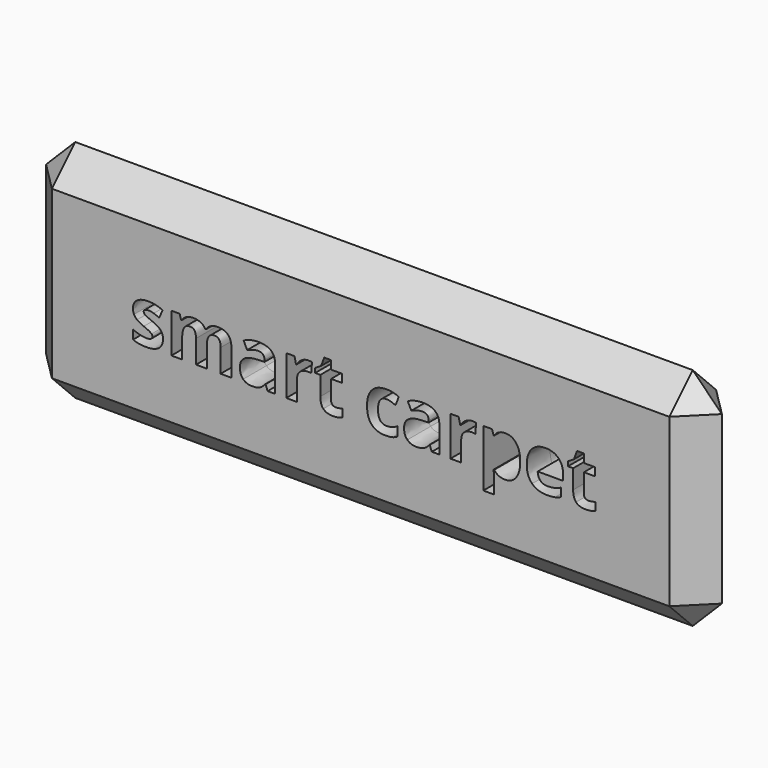
from build123d import *

# Parameters (mm, degrees)
F0_W     = 115.5963391066
F0_H     = 38.5321122594
F1_DEPTH = 5
F2_SIZE  = 4.99999


# Not quite as in the source:
# - a fillet or chamfer is up to 0.001 mm smaller than in the source, because OpenCascade refuses the exact size


with BuildPart() as f1:
    # F0 (on Front) → F1 (new body, symmetric)
    with BuildSketch(Plane.XZ):
        with Locations((0, 2.1674314048)):
            Rectangle(F0_W, F0_H)
        with BuildLine():
            add(Edge.make_bspline(
                [(-33.978614819, 0.8299154837), (-33.8024505908, 0.4669397388), (-33.8024505908, -0.0344507568)],
                knots=[0, 0, 0, 1, 1, 1], degree=2))
            add(Edge.make_bspline(
                [(-33.8024505908, -0.0344507568), (-33.8024505908, -1.0759491607), (-34.5254982746, -1.6208967457)],
                knots=[0, 0, 0, 1, 1, 1], degree=2))
            add(Edge.make_bspline(
                [(-34.5254982746, -1.6208967457), (-35.2485459583, -2.1658443306), (-36.688833714, -2.1658443306)],
                knots=[0, 0, 0, 1, 1, 1], degree=2))
            add(Edge.make_bspline(
                [(-36.688833714, -2.1658443306), (-37.4264004275, -2.1658443306), (-37.9471496295, -2.0651790574)],
                knots=[0, 0, 0, 1, 1, 1], degree=2))
            add(Edge.make_bspline(
                [(-37.9471496295, -2.0651790574), (-38.4678988315, -1.9645137842), (-38.9208925611, -1.7709267202)],
                knots=[0, 0, 0, 1, 1, 1], degree=2))
            Line((-38.9208925611, -1.7709267202), (-38.9208925611, -0.2473965271))
            add(Edge.make_bspline(
                [(-38.9208925611, -0.2473965271), (-38.4078868417, -0.489380357), (-37.7632419188, -0.652961426)],
                knots=[0, 0, 0, 1, 1, 1], degree=2))
            add(Edge.make_bspline(
                [(-37.7632419188, -0.652961426), (-37.1185969959, -0.8165424951), (-36.6288217242, -0.8165424951)],
                knots=[0, 0, 0, 1, 1, 1], degree=2))
            add(Edge.make_bspline(
                [(-36.6288217242, -0.8165424951), (-35.6241048624, -0.8165424951), (-35.6241048624, -0.2357813033)],
                knots=[0, 0, 0, 1, 1, 1], degree=2))
            add(Edge.make_bspline(
                [(-35.6241048624, -0.2357813033), (-35.6241048624, -0.017027921), (-35.7576799365, 0.119450959)],
                knots=[0, 0, 0, 1, 1, 1], degree=2))
            add(Edge.make_bspline(
                [(-35.7576799365, 0.119450959), (-35.8912550106, 0.2559298391), (-36.2174492133, 0.428222326)],
                knots=[0, 0, 0, 1, 1, 1], degree=2))
            add(Edge.make_bspline(
                [(-36.2174492133, 0.428222326), (-36.543643416, 0.6005148129), (-37.0876230657, 0.8289475483)],
                knots=[0, 0, 0, 1, 1, 1], degree=2))
            add(Edge.make_bspline(
                [(-37.0876230657, 0.8289475483), (-37.8677789333, 1.1561096864), (-38.2346264195, 1.4348750584)],
                knots=[0, 0, 0, 1, 1, 1], degree=2))
            add(Edge.make_bspline(
                [(-38.2346264195, 1.4348750584), (-38.6014739056, 1.7136404305), (-38.7669908453, 2.0737123694)],
                knots=[0, 0, 0, 1, 1, 1], degree=2))
            add(Edge.make_bspline(
                [(-38.7669908453, 2.0737123694), (-38.9325077849, 2.4337843083), (-38.9325077849, 2.9584052516)],
                knots=[0, 0, 0, 1, 1, 1], degree=2))
            add(Edge.make_bspline(
                [(-38.9325077849, 2.9584052516), (-38.9325077849, 3.8605209695), (-38.2346264195, 4.3532000472)],
                knots=[0, 0, 0, 1, 1, 1], degree=2))
            add(Edge.make_bspline(
                [(-38.2346264195, 4.3532000472), (-37.536745054, 4.8458791249), (-36.2532628201, 4.8458791249)],
                knots=[0, 0, 0, 1, 1, 1], degree=2))
            add(Edge.make_bspline(
                [(-36.2532628201, 4.8458791249), (-35.0317284467, 4.8458791249), (-33.8760136751, 4.3135146991)],
                knots=[0, 0, 0, 1, 1, 1], degree=2))
            Line((-33.8760136751, 4.3135146991), (-34.4316085486, 2.9835715699))
            add(Edge.make_bspline(
                [(-34.4316085486, 2.9835715699), (-34.9407425267, 3.2003890815), (-35.3821210324, 3.3397717675)],
                knots=[0, 0, 0, 1, 1, 1], degree=2))
            add(Edge.make_bspline(
                [(-35.3821210324, 3.3397717675), (-35.8234995382, 3.4791544535), (-36.2842367504, 3.4791544535)],
                knots=[0, 0, 0, 1, 1, 1], degree=2))
            add(Edge.make_bspline(
                [(-36.2842367504, 3.4791544535), (-37.1011741601, 3.4791544535), (-37.1011741601, 3.0377759478)],
                knots=[0, 0, 0, 1, 1, 1], degree=2))
            add(Edge.make_bspline(
                [(-37.1011741601, 3.0377759478), (-37.1011741601, 2.789984506), (-36.8378957532, 2.6080126659)],
                knots=[0, 0, 0, 1, 1, 1], degree=2))
            add(Edge.make_bspline(
                [(-36.8378957532, 2.6080126659), (-36.5746173463, 2.4260408258), (-35.6841168522, 2.0698406281)],
                knots=[0, 0, 0, 1, 1, 1], degree=2))
            add(Edge.make_bspline(
                [(-35.6841168522, 2.0698406281), (-34.8923457607, 1.748486102), (-34.5235624039, 1.4706886653)],
                knots=[0, 0, 0, 1, 1, 1], degree=2))
            add(Edge.make_bspline(
                [(-34.5235624039, 1.4706886653), (-34.1547790471, 1.1928912285), (-33.978614819, 0.8299154837)],
                knots=[0, 0, 0, 1, 1, 1], degree=2))
        make_face(mode=Mode.SUBTRACT)
        with BuildLine():
            Line((-26.3086953461, 1.3496967503), (-26.3086953461, -2.0438844804))
            Line((-26.3086953461, -2.0438844804), (-28.1535800653, -2.0438844804))
            Line((-28.1535800653, -2.0438844804), (-28.1535800653, 1.9072274944))
            add(Edge.make_bspline(
                [(-28.1535800653, 1.9072274944), (-28.1535800653, 2.6389865961), (-28.3984677012, 3.0048661469)],
                knots=[0, 0, 0, 1, 1, 1], degree=2))
            add(Edge.make_bspline(
                [(-28.3984677012, 3.0048661469), (-28.6433553371, 3.3707456977), (-29.1699121509, 3.3707456977)],
                knots=[0, 0, 0, 1, 1, 1], degree=2))
            add(Edge.make_bspline(
                [(-29.1699121509, 3.3707456977), (-29.8784408049, 3.3707456977), (-30.1988273957, 2.8499964958)],
                knots=[0, 0, 0, 1, 1, 1], degree=2))
            add(Edge.make_bspline(
                [(-30.1988273957, 2.8499964958), (-30.5192139865, 2.3292472938), (-30.5192139865, 1.1386868506)],
                knots=[0, 0, 0, 1, 1, 1], degree=2))
            Line((-30.5192139865, 1.1386868506), (-30.5192139865, -2.0438844804))
            Line((-30.5192139865, -2.0438844804), (-32.3640987058, -2.0438844804))
            Line((-32.3640987058, -2.0438844804), (-32.3640987058, 4.7200475333))
            Line((-32.3640987058, 4.7200475333), (-30.9547848804, 4.7200475333))
            Line((-30.9547848804, 4.7200475333), (-30.7069934385, 3.8547133576))
            Line((-30.7069934385, 3.8547133576), (-30.6043922947, 3.8547133576))
            add(Edge.make_bspline(
                [(-30.6043922947, 3.8547133576), (-30.3314345345, 4.3212581816), (-29.8174608798, 4.5835686533)],
                knots=[0, 0, 0, 1, 1, 1], degree=2))
            add(Edge.make_bspline(
                [(-29.8174608798, 4.5835686533), (-29.3034872251, 4.8458791249), (-28.6375477251, 4.8458791249)],
                knots=[0, 0, 0, 1, 1, 1], degree=2))
            add(Edge.make_bspline(
                [(-28.6375477251, 4.8458791249), (-27.1198251439, 4.8458791249), (-26.5797172356, 3.8547133576)],
                knots=[0, 0, 0, 1, 1, 1], degree=2))
            Line((-26.5797172356, 3.8547133576), (-26.4171041019, 3.8547133576))
            add(Edge.make_bspline(
                [(-26.4171041019, 3.8547133576), (-26.1441463417, 4.3270657936), (-25.6156536572, 4.5864724592)],
                knots=[0, 0, 0, 1, 1, 1], degree=2))
            add(Edge.make_bspline(
                [(-25.6156536572, 4.5864724592), (-25.0871609727, 4.8458791249), (-24.4212214727, 4.8458791249)],
                knots=[0, 0, 0, 1, 1, 1], degree=2))
            add(Edge.make_bspline(
                [(-24.4212214727, 4.8458791249), (-23.271314313, 4.8458791249), (-22.6818417033, 4.2564065152)],
                knots=[0, 0, 0, 1, 1, 1], degree=2))
            add(Edge.make_bspline(
                [(-22.6818417033, 4.2564065152), (-22.0923690937, 3.6669339056), (-22.0923690937, 2.3660288359)],
                knots=[0, 0, 0, 1, 1, 1], degree=2))
            Line((-22.0923690937, 2.3660288359), (-22.0923690937, -2.0438844804))
            Line((-22.0923690937, -2.0438844804), (-23.9430614248, -2.0438844804))
            Line((-23.9430614248, -2.0438844804), (-23.9430614248, 1.9072274944))
            add(Edge.make_bspline(
                [(-23.9430614248, 1.9072274944), (-23.9430614248, 2.6389865961), (-24.1879490607, 3.0048661469)],
                knots=[0, 0, 0, 1, 1, 1], degree=2))
            add(Edge.make_bspline(
                [(-24.1879490607, 3.0048661469), (-24.4328366966, 3.3707456977), (-24.9593935105, 3.3707456977)],
                knots=[0, 0, 0, 1, 1, 1], degree=2))
            add(Edge.make_bspline(
                [(-24.9593935105, 3.3707456977), (-25.6369482342, 3.3707456977), (-25.9728217901, 2.8867780379)],
                knots=[0, 0, 0, 1, 1, 1], degree=2))
            add(Edge.make_bspline(
                [(-25.9728217901, 2.8867780379), (-26.3086953461, 2.4028103781), (-26.3086953461, 1.3496967503)],
                knots=[0, 0, 0, 1, 1, 1], degree=2))
        make_face(mode=Mode.SUBTRACT)
        with BuildLine():
            Line((-14.6160366847, -2.0438844804), (-15.9033906598, -2.0438844804))
            Line((-15.9033906598, -2.0438844804), (-16.2615267281, -1.1243459267))
            Line((-16.2615267281, -1.1243459267), (-16.3099234941, -1.1243459267))
            add(Edge.make_bspline(
                [(-16.3099234941, -1.1243459267), (-16.7745324475, -1.7109147304), (-17.2681794605, -1.9383795305)],
                knots=[0, 0, 0, 1, 1, 1], degree=2))
            add(Edge.make_bspline(
                [(-17.2681794605, -1.9383795305), (-17.7618264736, -2.1658443306), (-18.553597565, -2.1658443306)],
                knots=[0, 0, 0, 1, 1, 1], degree=2))
            add(Edge.make_bspline(
                [(-18.553597565, -2.1658443306), (-19.5273404966, -2.1658443306), (-20.0868071114, -1.6083135865)],
                knots=[0, 0, 0, 1, 1, 1], degree=2))
            add(Edge.make_bspline(
                [(-20.0868071114, -1.6083135865), (-20.6462737261, -1.0507828424), (-20.6462737261, -0.0228355329)],
                knots=[0, 0, 0, 1, 1, 1], degree=2))
            add(Edge.make_bspline(
                [(-20.6462737261, -0.0228355329), (-20.6462737261, 1.0535085425), (-19.8932200474, 1.5645783913)],
                knots=[0, 0, 0, 1, 1, 1], degree=2))
            add(Edge.make_bspline(
                [(-19.8932200474, 1.5645783913), (-19.1401663687, 2.0756482401), (-17.6224437875, 2.129852618)],
                knots=[0, 0, 0, 1, 1, 1], degree=2))
            Line((-17.6224437875, 2.129852618), (-16.4473703095, 2.1666341601))
            Line((-16.4473703095, 2.1666341601), (-16.4473703095, 2.4628223679))
            add(Edge.make_bspline(
                [(-16.4473703095, 2.4628223679), (-16.4473703095, 3.4907696774), (-17.5004839373, 3.4907696774)],
                knots=[0, 0, 0, 1, 1, 1], degree=2))
            add(Edge.make_bspline(
                [(-17.5004839373, 3.4907696774), (-18.3116137351, 3.4907696774), (-19.407316517, 3.0009944056)],
                knots=[0, 0, 0, 1, 1, 1], degree=2))
            Line((-19.407316517, 3.0009944056), (-20.0171157683, 4.2476950973))
            add(Edge.make_bspline(
                [(-20.0171157683, 4.2476950973), (-18.8497857728, 4.8594302194), (-17.4288567236, 4.8594302194)],
                knots=[0, 0, 0, 1, 1, 1], degree=2))
            add(Edge.make_bspline(
                [(-17.4288567236, 4.8594302194), (-16.0679396642, 4.8594302194), (-15.3419881744, 4.2660858684)],
                knots=[0, 0, 0, 1, 1, 1], degree=2))
            add(Edge.make_bspline(
                [(-15.3419881744, 4.2660858684), (-14.6160366847, 3.6727415175), (-14.6160366847, 2.4628223679)],
                knots=[0, 0, 0, 1, 1, 1], degree=2))
            Line((-14.6160366847, 2.4628223679), (-14.6160366847, -2.0438844804))
        make_face(mode=Mode.SUBTRACT)
        with BuildLine():
            add(Edge.make_bspline(
                [(-10.1044901598, 4.4983903451), (-9.5692219281, 4.8458791249), (-8.9400639703, 4.8458791249)],
                knots=[0, 0, 0, 1, 1, 1], degree=2))
            add(Edge.make_bspline(
                [(-8.9400639703, 4.8458791249), (-8.5645050663, 4.8458791249), (-8.3167136244, 4.791674747)],
                knots=[0, 0, 0, 1, 1, 1], degree=2))
            Line((-8.3167136244, 4.791674747), (-8.4560963105, 3.0629422661))
            add(Edge.make_bspline(
                [(-8.4560963105, 3.0629422661), (-8.6806573046, 3.1229542559), (-9.0000759601, 3.1229542559)],
                knots=[0, 0, 0, 1, 1, 1], degree=2))
            add(Edge.make_bspline(
                [(-9.0000759601, 3.1229542559), (-9.8828329716, 3.1229542559), (-10.3764799846, 2.668992591)],
                knots=[0, 0, 0, 1, 1, 1], degree=2))
            add(Edge.make_bspline(
                [(-10.3764799846, 2.668992591), (-10.8701269977, 2.2150309261), (-10.8701269977, 1.3980935163)],
                knots=[0, 0, 0, 1, 1, 1], degree=2))
            Line((-10.8701269977, 1.3980935163), (-10.8701269977, -2.0438844804))
            Line((-10.8701269977, -2.0438844804), (-12.7150117169, -2.0438844804))
            Line((-12.7150117169, -2.0438844804), (-12.7150117169, 4.7200475333))
            Line((-12.7150117169, 4.7200475333), (-11.3173131153, 4.7200475333))
            Line((-11.3173131153, 4.7200475333), (-11.0443553552, 3.5817555974))
            Line((-11.0443553552, 3.5817555974), (-10.9553053058, 3.5817555974))
            add(Edge.make_bspline(
                [(-10.9553053058, 3.5817555974), (-10.6397583916, 4.1509015654), (-10.1044901598, 4.4983903451)],
                knots=[0, 0, 0, 1, 1, 1], degree=2))
        make_face(mode=Mode.SUBTRACT)
        with BuildLine():
            add(Edge.make_bspline(
                [(-4.8244029911, -0.5068031928), (-4.6037137383, -0.6945826448), (-4.2397700581, -0.6945826448)],
                knots=[0, 0, 0, 1, 1, 1], degree=2))
            add(Edge.make_bspline(
                [(-4.2397700581, -0.6945826448), (-3.7558023982, -0.6945826448), (-3.0782476745, -0.4835727451)],
                knots=[0, 0, 0, 1, 1, 1], degree=2))
            Line((-3.0782476745, -0.4835727451), (-3.0782476745, -1.8561050284))
            add(Edge.make_bspline(
                [(-3.0782476745, -1.8561050284), (-3.7674176221, -2.1658443306), (-4.7721344839, -2.1658443306)],
                knots=[0, 0, 0, 1, 1, 1], degree=2))
            add(Edge.make_bspline(
                [(-4.7721344839, -2.1658443306), (-5.8794524896, -2.1658443306), (-6.3847147264, -1.6054097806)],
                knots=[0, 0, 0, 1, 1, 1], degree=2))
            add(Edge.make_bspline(
                [(-6.3847147264, -1.6054097806), (-6.8899769633, -1.0449752305), (-6.8899769633, 0.073957999)],
                knots=[0, 0, 0, 1, 1, 1], degree=2))
            Line((-6.8899769633, 0.073957999), (-6.8899769633, 3.3339641556))
            Line((-6.8899769633, 3.3339641556), (-7.7727339748, 3.3339641556))
            Line((-7.7727339748, 3.3339641556), (-7.7727339748, 4.1141200232))
            Line((-7.7727339748, 4.1141200232), (-6.7564018892, 4.7316627572))
            Line((-6.7564018892, 4.7316627572), (-6.2240374633, 6.160335289))
            Line((-6.2240374633, 6.160335289), (-5.045092244, 6.160335289))
            Line((-5.045092244, 6.160335289), (-5.045092244, 4.7200475333))
            Line((-5.045092244, 4.7200475333), (-3.1518107588, 4.7200475333))
            Line((-3.1518107588, 4.7200475333), (-3.1518107588, 3.3339641556))
            Line((-3.1518107588, 3.3339641556), (-5.045092244, 3.3339641556))
            Line((-5.045092244, 3.3339641556), (-5.045092244, 0.073957999))
            add(Edge.make_bspline(
                [(-5.045092244, 0.073957999), (-5.045092244, -0.3190237408), (-4.8244029911, -0.5068031928)],
                knots=[0, 0, 0, 1, 1, 1], degree=2))
        make_face(mode=Mode.SUBTRACT)
        with BuildLine():
            add(Edge.make_bspline(
                [(5.4066733375, -2.0564676395), (4.9498078667, -2.1658443306), (4.2548303072, -2.1658443306)],
                knots=[0, 0, 0, 1, 1, 1], degree=2))
            add(Edge.make_bspline(
                [(4.2548303072, -2.1658443306), (1.0974252945, -2.1658443306), (1.0974252945, 1.3012999843)],
                knots=[0, 0, 0, 1, 1, 1], degree=2))
            add(Edge.make_bspline(
                [(1.0974252945, 1.3012999843), (1.0974252945, 3.0261607239), (1.955983923, 3.9360199244)],
                knots=[0, 0, 0, 1, 1, 1], degree=2))
            add(Edge.make_bspline(
                [(1.955983923, 3.9360199244), (2.8145425515, 4.8458791249), (4.4174434409, 4.8458791249)],
                knots=[0, 0, 0, 1, 1, 1], degree=2))
            add(Edge.make_bspline(
                [(4.4174434409, 4.8458791249), (5.5905810483, 4.8458791249), (6.5236706964, 4.3870777834)],
                knots=[0, 0, 0, 1, 1, 1], degree=2))
            Line((6.5236706964, 4.3870777834), (5.9777551761, 2.9584052516))
            add(Edge.make_bspline(
                [(5.9777551761, 2.9584052516), (5.5421842823, 3.1345694797), (5.1675933136, 3.2468499768)],
                knots=[0, 0, 0, 1, 1, 1], degree=2))
            add(Edge.make_bspline(
                [(5.1675933136, 3.2468499768), (4.7930023449, 3.3591304739), (4.4174434409, 3.3591304739)],
                knots=[0, 0, 0, 1, 1, 1], degree=2))
            add(Edge.make_bspline(
                [(4.4174434409, 3.3591304739), (2.9771556852, 3.3591304739), (2.9771556852, 1.3129152082)],
                knots=[0, 0, 0, 1, 1, 1], degree=2))
            add(Edge.make_bspline(
                [(2.9771556852, 1.3129152082), (2.9771556852, -0.6713521971), (4.4174434409, -0.6713521971)],
                knots=[0, 0, 0, 1, 1, 1], degree=2))
            add(Edge.make_bspline(
                [(4.4174434409, -0.6713521971), (4.9498078667, -0.6713521971), (5.4037695316, -0.5290657051)],
                knots=[0, 0, 0, 1, 1, 1], degree=2))
            add(Edge.make_bspline(
                [(5.4037695316, -0.5290657051), (5.8577311965, -0.3867792131), (6.3107249261, -0.0828475228)],
                knots=[0, 0, 0, 1, 1, 1], degree=2))
            Line((6.3107249261, -0.0828475228), (6.3107249261, -1.6625179644))
            add(Edge.make_bspline(
                [(6.3107249261, -1.6625179644), (5.8635388084, -1.9470909484), (5.4066733375, -2.0564676395)],
                knots=[0, 0, 0, 1, 1, 1], degree=2))
        make_face(mode=Mode.SUBTRACT)
        with BuildLine():
            Line((13.4618310677, -2.0438844804), (12.1744770925, -2.0438844804))
            Line((12.1744770925, -2.0438844804), (11.8163410243, -1.1243459267))
            Line((11.8163410243, -1.1243459267), (11.7679442583, -1.1243459267))
            add(Edge.make_bspline(
                [(11.7679442583, -1.1243459267), (11.3033353048, -1.7109147304), (10.8096882918, -1.9383795305)],
                knots=[0, 0, 0, 1, 1, 1], degree=2))
            add(Edge.make_bspline(
                [(10.8096882918, -1.9383795305), (10.3160412788, -2.1658443306), (9.5242701873, -2.1658443306)],
                knots=[0, 0, 0, 1, 1, 1], degree=2))
            add(Edge.make_bspline(
                [(9.5242701873, -2.1658443306), (8.5505272558, -2.1658443306), (7.991060641, -1.6083135865)],
                knots=[0, 0, 0, 1, 1, 1], degree=2))
            add(Edge.make_bspline(
                [(7.991060641, -1.6083135865), (7.4315940263, -1.0507828424), (7.4315940263, -0.0228355329)],
                knots=[0, 0, 0, 1, 1, 1], degree=2))
            add(Edge.make_bspline(
                [(7.4315940263, -0.0228355329), (7.4315940263, 1.0535085425), (8.1846477049, 1.5645783913)],
                knots=[0, 0, 0, 1, 1, 1], degree=2))
            add(Edge.make_bspline(
                [(8.1846477049, 1.5645783913), (8.9377013836, 2.0756482401), (10.4554239648, 2.129852618)],
                knots=[0, 0, 0, 1, 1, 1], degree=2))
            Line((10.4554239648, 2.129852618), (11.6304974429, 2.1666341601))
            Line((11.6304974429, 2.1666341601), (11.6304974429, 2.4628223679))
            add(Edge.make_bspline(
                [(11.6304974429, 2.4628223679), (11.6304974429, 3.4907696774), (10.5773838151, 3.4907696774)],
                knots=[0, 0, 0, 1, 1, 1], degree=2))
            add(Edge.make_bspline(
                [(10.5773838151, 3.4907696774), (9.7662540172, 3.4907696774), (8.6705512354, 3.0009944056)],
                knots=[0, 0, 0, 1, 1, 1], degree=2))
            Line((8.6705512354, 3.0009944056), (8.060751984, 4.2476950973))
            add(Edge.make_bspline(
                [(8.060751984, 4.2476950973), (9.2280819795, 4.8594302194), (10.6490110288, 4.8594302194)],
                knots=[0, 0, 0, 1, 1, 1], degree=2))
            add(Edge.make_bspline(
                [(10.6490110288, 4.8594302194), (12.0099280882, 4.8594302194), (12.7358795779, 4.2660858684)],
                knots=[0, 0, 0, 1, 1, 1], degree=2))
            add(Edge.make_bspline(
                [(12.7358795779, 4.2660858684), (13.4618310677, 3.6727415175), (13.4618310677, 2.4628223679)],
                knots=[0, 0, 0, 1, 1, 1], degree=2))
            Line((13.4618310677, 2.4628223679), (13.4618310677, -2.0438844804))
        make_face(mode=Mode.SUBTRACT)
        with BuildLine():
            add(Edge.make_bspline(
                [(17.9733775925, 4.4983903451), (18.5086458243, 4.8458791249), (19.1378037821, 4.8458791249)],
                knots=[0, 0, 0, 1, 1, 1], degree=2))
            add(Edge.make_bspline(
                [(19.1378037821, 4.8458791249), (19.5133626861, 4.8458791249), (19.7611541279, 4.791674747)],
                knots=[0, 0, 0, 1, 1, 1], degree=2))
            Line((19.7611541279, 4.791674747), (19.6217714419, 3.0629422661))
            add(Edge.make_bspline(
                [(19.6217714419, 3.0629422661), (19.3972104478, 3.1229542559), (19.0777917923, 3.1229542559)],
                knots=[0, 0, 0, 1, 1, 1], degree=2))
            add(Edge.make_bspline(
                [(19.0777917923, 3.1229542559), (18.1950347807, 3.1229542559), (17.7013877677, 2.668992591)],
                knots=[0, 0, 0, 1, 1, 1], degree=2))
            add(Edge.make_bspline(
                [(17.7013877677, 2.668992591), (17.2077407547, 2.2150309261), (17.2077407547, 1.3980935163)],
                knots=[0, 0, 0, 1, 1, 1], degree=2))
            Line((17.2077407547, 1.3980935163), (17.2077407547, -2.0438844804))
            Line((17.2077407547, -2.0438844804), (15.3628560355, -2.0438844804))
            Line((15.3628560355, -2.0438844804), (15.3628560355, 4.7200475333))
            Line((15.3628560355, 4.7200475333), (16.760554637, 4.7200475333))
            Line((16.760554637, 4.7200475333), (17.0335123972, 3.5817555974))
            Line((17.0335123972, 3.5817555974), (17.1225624466, 3.5817555974))
            add(Edge.make_bspline(
                [(17.1225624466, 3.5817555974), (17.4381093608, 4.1509015654), (17.9733775925, 4.4983903451)],
                knots=[0, 0, 0, 1, 1, 1], degree=2))
        make_face(mode=Mode.SUBTRACT)
        with BuildLine():
            add(Edge.make_bspline(
                [(26.0817717652, -1.7476962726), (25.4952029615, -2.1658443306), (24.7034318701, -2.1658443306)],
                knots=[0, 0, 0, 1, 1, 1], degree=2))
            add(Edge.make_bspline(
                [(24.7034318701, -2.1658443306), (23.5109355563, -2.1658443306), (22.8333808325, -1.3005101549)],
                knots=[0, 0, 0, 1, 1, 1], degree=2))
            Line((22.8333808325, -1.3005101549), (22.7365873005, -1.3005101549))
            add(Edge.make_bspline(
                [(22.7365873005, -1.3005101549), (22.8333808325, -2.1464856243), (22.8333808325, -2.2800606984)],
                knots=[0, 0, 0, 1, 1, 1], degree=2))
            Line((22.8333808325, -2.2800606984), (22.8333808325, -5.0212535236))
            Line((22.8333808325, -5.0212535236), (20.9884961133, -5.0212535236))
            Line((20.9884961133, -5.0212535236), (20.9884961133, 4.7200475333))
            Line((20.9884961133, 4.7200475333), (22.4887958587, 4.7200475333))
            Line((22.4887958587, 4.7200475333), (22.7482025244, 3.8430981337))
            Line((22.7482025244, 3.8430981337), (22.8333808325, 3.8430981337))
            add(Edge.make_bspline(
                [(22.8333808325, 3.8430981337), (23.4818974967, 4.8458791249), (24.751828636, 4.8458791249)],
                knots=[0, 0, 0, 1, 1, 1], degree=2))
            add(Edge.make_bspline(
                [(24.751828636, 4.8458791249), (25.9501325618, 4.8458791249), (26.6276872855, 3.9205329593)],
                knots=[0, 0, 0, 1, 1, 1], degree=2))
            add(Edge.make_bspline(
                [(26.6276872855, 3.9205329593), (27.3052420093, 2.9951867937), (27.3052420093, 1.3496967503)],
                knots=[0, 0, 0, 1, 1, 1], degree=2))
            add(Edge.make_bspline(
                [(27.3052420093, 1.3496967503), (27.3052420093, 0.2675450629), (26.9867912891, -0.5310015758)],
                knots=[0, 0, 0, 1, 1, 1], degree=2))
            add(Edge.make_bspline(
                [(26.9867912891, -0.5310015758), (26.668340569, -1.3295482145), (26.0817717652, -1.7476962726)],
                knots=[0, 0, 0, 1, 1, 1], degree=2))
        make_face(mode=Mode.SUBTRACT)
        with BuildLine():
            add(Edge.make_bspline(
                [(33.2328779068, -2.0477562217), (32.6830906453, -2.1658443306), (31.8893836831, -2.1658443306)],
                knots=[0, 0, 0, 1, 1, 1], degree=2))
            add(Edge.make_bspline(
                [(31.8893836831, -2.1658443306), (30.2574447342, -2.1658443306), (29.3379061805, -1.2637286127)],
                knots=[0, 0, 0, 1, 1, 1], degree=2))
            add(Edge.make_bspline(
                [(29.3379061805, -1.2637286127), (28.4183676269, -0.3616128948), (28.4183676269, 1.2896847605)],
                knots=[0, 0, 0, 1, 1, 1], degree=2))
            add(Edge.make_bspline(
                [(28.4183676269, 1.2896847605), (28.4183676269, 2.9893791818), (29.2682148375, 3.9176291533)],
                knots=[0, 0, 0, 1, 1, 1], degree=2))
            add(Edge.make_bspline(
                [(29.2682148375, 3.9176291533), (30.1180620482, 4.8458791249), (31.6183617936, 4.8458791249)],
                knots=[0, 0, 0, 1, 1, 1], degree=2))
            add(Edge.make_bspline(
                [(31.6183617936, 4.8458791249), (33.0509060667, 4.8458791249), (33.8494527054, 4.0299096504)],
                knots=[0, 0, 0, 1, 1, 1], degree=2))
            add(Edge.make_bspline(
                [(33.8494527054, 4.0299096504), (34.6479993441, 3.213940176), (34.6479993441, 1.7736524203)],
                knots=[0, 0, 0, 1, 1, 1], degree=2))
            Line((34.6479993441, 1.7736524203), (34.6479993441, 0.8773443143))
            Line((34.6479993441, 0.8773443143), (30.2864827938, 0.8773443143))
            add(Edge.make_bspline(
                [(30.2864827938, 0.8773443143), (30.317456724, 0.0913808348), (30.7530276179, -0.349997671)],
                knots=[0, 0, 0, 1, 1, 1], degree=2))
            add(Edge.make_bspline(
                [(30.7530276179, -0.349997671), (31.1885985117, -0.7913761767), (31.9745619913, -0.7913761767)],
                knots=[0, 0, 0, 1, 1, 1], degree=2))
            add(Edge.make_bspline(
                [(31.9745619913, -0.7913761767), (32.5862971133, -0.7913761767), (33.1302767629, -0.6645766499)],
                knots=[0, 0, 0, 1, 1, 1], degree=2))
            add(Edge.make_bspline(
                [(33.1302767629, -0.6645766499), (33.6742564126, -0.537777123), (34.2666328282, -0.2590117509)],
                knots=[0, 0, 0, 1, 1, 1], degree=2))
            Line((34.2666328282, -0.2590117509), (34.2666328282, -1.6876842827))
            add(Edge.make_bspline(
                [(34.2666328282, -1.6876842827), (33.7826651684, -1.9296681127), (33.2328779068, -2.0477562217)],
                knots=[0, 0, 0, 1, 1, 1], degree=2))
        make_face(mode=Mode.SUBTRACT)
        with BuildLine():
            add(Edge.make_bspline(
                [(38.4132677376, -0.5068031928), (38.6339569905, -0.6945826448), (38.9979006706, -0.6945826448)],
                knots=[0, 0, 0, 1, 1, 1], degree=2))
            add(Edge.make_bspline(
                [(38.9979006706, -0.6945826448), (39.4818683305, -0.6945826448), (40.1594230542, -0.4835727451)],
                knots=[0, 0, 0, 1, 1, 1], degree=2))
            Line((40.1594230542, -0.4835727451), (40.1594230542, -1.8561050284))
            add(Edge.make_bspline(
                [(40.1594230542, -1.8561050284), (39.4702531066, -2.1658443306), (38.4655362448, -2.1658443306)],
                knots=[0, 0, 0, 1, 1, 1], degree=2))
            add(Edge.make_bspline(
                [(38.4655362448, -2.1658443306), (37.3582182392, -2.1658443306), (36.8529560023, -1.6054097806)],
                knots=[0, 0, 0, 1, 1, 1], degree=2))
            add(Edge.make_bspline(
                [(36.8529560023, -1.6054097806), (36.3476937654, -1.0449752305), (36.3476937654, 0.073957999)],
                knots=[0, 0, 0, 1, 1, 1], degree=2))
            Line((36.3476937654, 0.073957999), (36.3476937654, 3.3339641556))
            Line((36.3476937654, 3.3339641556), (35.4649367539, 3.3339641556))
            Line((35.4649367539, 3.3339641556), (35.4649367539, 4.1141200232))
            Line((35.4649367539, 4.1141200232), (36.4812688396, 4.7316627572))
            Line((36.4812688396, 4.7316627572), (37.0136332654, 6.160335289))
            Line((37.0136332654, 6.160335289), (38.1925784847, 6.160335289))
            Line((38.1925784847, 6.160335289), (38.1925784847, 4.7200475333))
            Line((38.1925784847, 4.7200475333), (40.0858599699, 4.7200475333))
            Line((40.0858599699, 4.7200475333), (40.0858599699, 3.3339641556))
            Line((40.0858599699, 3.3339641556), (38.1925784847, 3.3339641556))
            Line((38.1925784847, 3.3339641556), (38.1925784847, 0.073957999))
            add(Edge.make_bspline(
                [(38.1925784847, 0.073957999), (38.1925784847, -0.3190237408), (38.4132677376, -0.5068031928)],
                knots=[0, 0, 0, 1, 1, 1], degree=2))
        make_face(mode=Mode.SUBTRACT)
    extrude(amount=F1_DEPTH, both=True)

    # F2 (size 5 in the source; OpenCascade refuses exactly that, so slightly less here)
    f2_edges = [f1.edges().sort_by_distance(p)[0] for p in [
        (57.79817, 5, 2.167431),
        (57.79817, 0, 21.433488),
        (57.79817, -5, 2.167431),
        (57.79817, 0, -17.098625),
        (-57.79817, 0, -17.098625),
        (0, 5, -17.098625),
        (0, -5, -17.098625),
        (0, 5, 21.433488),
        (-57.79817, 0, 21.433488),
        (0, -5, 21.433488),
        (-57.79817, 5, 2.167431),
        (-57.79817, -5, 2.167431),
    ]]
    chamfer(f2_edges, length=F2_SIZE)


solid = f1.part
